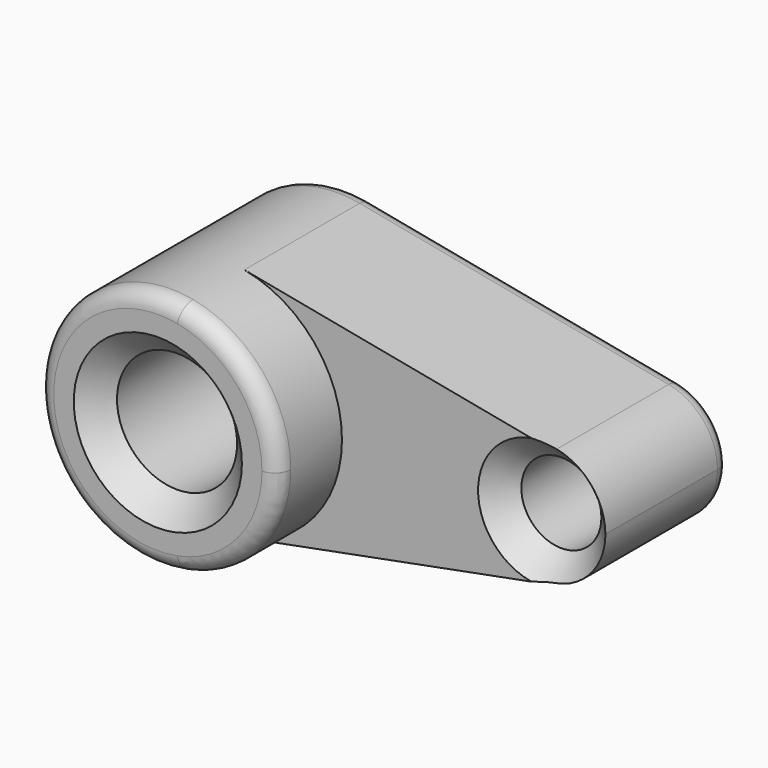
from build123d import *

# Parameters (mm, degrees)
F0_R     = 9.525
F0_R_2   = 6.35
F1_DEPTH = 25.4
F2_DEPTH = 38.1
F3_R     = 2.54


# Not quite as in the source:
# - a fillet or chamfer that OpenCascade refuses, or shapes differently, is made with other operations: its cross-section is extruded or revolved along the edge and cut away or added


with BuildPart() as f1:
    # F0 (on Front) → F1 (new body)
    with BuildSketch(Plane.XZ):
        with BuildLine():
            ThreePointArc((3.571875, -18.7121406842), (14.6790108446, -12.1420402167), (19.05, 0))
            ThreePointArc((19.05, 0), (14.6790108446, 12.1420402167), (3.571875, 18.7121406842))
            ThreePointArc((3.571875, 18.7121406842), (-19.05, 0), (3.571875, -18.7121406842))
        make_face()
        Circle(F0_R, mode=Mode.SUBTRACT)
        with BuildLine():
            ThreePointArc((3.571875, 18.7121406842), (14.6790108446, 12.1420402167), (19.05, 0))
            ThreePointArc((19.05, 0), (14.6790108446, -12.1420402167), (3.571875, -18.7121406842))
            Line((3.571875, -18.7121406842), (52.5859375, -9.3560703421))
            ThreePointArc((52.5859375, -9.3560703421), (41.275, 0), (52.5859375, 9.3560703421))
            Line((52.5859375, 9.3560703421), (3.571875, 18.7121406842))
        make_face()
        with BuildLine():
            ThreePointArc((60.325, 0), (58.1395054223, 6.0710201084), (52.5859375, 9.3560703421))
            ThreePointArc((52.5859375, 9.3560703421), (41.275, 0), (52.5859375, -9.3560703421))
            ThreePointArc((52.5859375, -9.3560703421), (58.1395054223, -6.0710201084), (60.325, 0))
        make_face()
        with Locations((50.8, 0)):
            Circle(F0_R_2, mode=Mode.SUBTRACT)
    extrude(amount=F1_DEPTH)

    # F0 (on Front) → F2 (join)
    with BuildSketch(Plane.XZ):
        with BuildLine():
            ThreePointArc((3.571875, -18.7121406842), (14.6790108446, -12.1420402167), (19.05, 0))
            ThreePointArc((19.05, 0), (14.6790108446, 12.1420402167), (3.571875, 18.7121406842))
            ThreePointArc((3.571875, 18.7121406842), (-19.05, 0), (3.571875, -18.7121406842))
        make_face()
        Circle(F0_R, mode=Mode.SUBTRACT)
    extrude(amount=F2_DEPTH)

    # F3
    f3_edges = [f1.edges().sort_by_distance(p)[0] for p in [
        (28.078906, 0, -14.034106),
        (-3.571875, -38.1, 18.712141),
    ]]
    fillet(f3_edges, radius=F3_R)

    # F4: chamfer of 3.81 on 4 edges, made by hand

    # F4_s1 → F4_t2 (revolve, cut)
    with BuildSketch(Plane.XY):
        Polygon((13.335, -38.1), (9.525, -34.29), (9.525, -38.1), align=None)
    revolve(axis=Axis((0, -38.1, 0), (0, -1, 0)), mode=Mode.SUBTRACT)

    # F4_s3 → F4_t4 (revolve, cut)
    with BuildSketch(Plane.XY):
        Polygon((60.96, -25.4), (57.15, -21.59), (57.15, -25.4), align=None)
    revolve(axis=Axis((50.8, -25.4, 0), (0, -1, 0)), mode=Mode.SUBTRACT)

    # F4_s5 → F4_t6 (revolve, cut)
    with BuildSketch(Plane.XY):
        Polygon((13.335, 0), (9.525, -3.81), (9.525, 0), align=None)
    revolve(axis=Axis((0, 0, 0), (0, -1, 0)), mode=Mode.SUBTRACT)

    # F4_s7 → F4_t8 (revolve, cut)
    with BuildSketch(Plane.XY):
        Polygon((60.96, 0), (57.15, -3.81), (57.15, 0), align=None)
    revolve(axis=Axis((50.8, 0, 0), (0, -1, 0)), mode=Mode.SUBTRACT)


solid = f1.part
